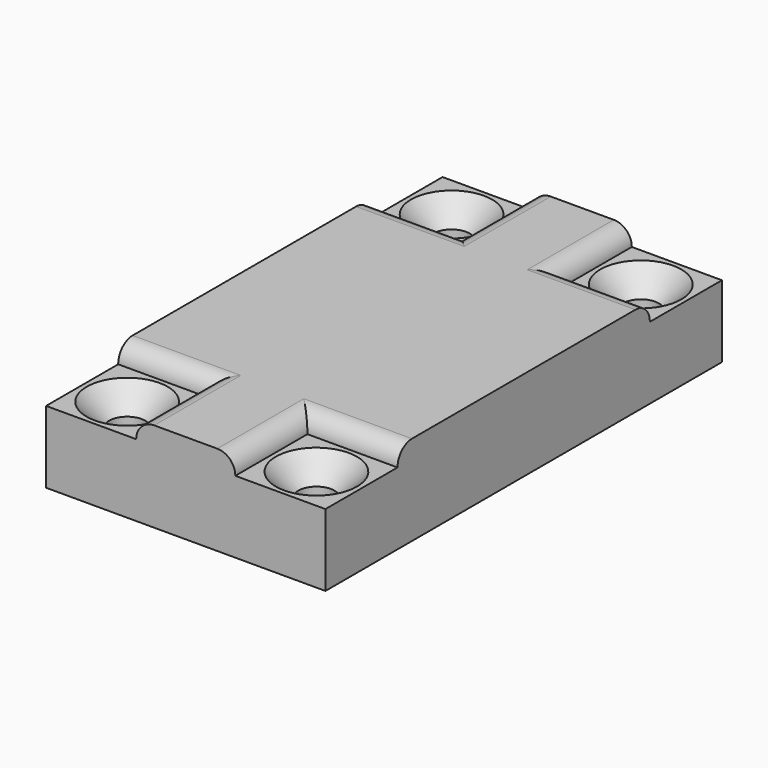
from build123d import *

# Parameters (mm, degrees)
F0_W     = 10
F0_H     = 18.5
F2_DEPTH = 10
F3_DEPTH = 3
F0_H_2   = 10
F4_DEPTH = 8
F1_R     = 2
F5_DEPTH = 25
F6_SIZE  = 2.5
F7_R     = 1.99999


# Not quite as in the source:
# - a fillet or chamfer is up to 0.001 mm smaller than in the source, because OpenCascade refuses the exact size


with BuildPart() as f2:
    # F0 (on Top) → F2 (new body)
    with BuildSketch(Plane.XY):
        with Locations((-10.5, 0.1457649022)):
            Rectangle(F0_W, F0_H)
        Polygon((5.5, 17.5), (5.5, 27.5), (-5.5, 27.5), (-5.5, 17.5), (-15.5, 17.5), (-15.5, 9.3957649022), (-5.5, 9.3957649022), (-5.5, -9.1042350978), (-15.5, -9.1042350978), (-15.5, -17.5), (-5.5, -17.5), (-5.5, -27.5), (5.5, -27.5), (5.5, -17.5), (15.5, -17.5), (15.5, 17.5), align=None)
    extrude(amount=F2_DEPTH)

    # F0 (on Top) → F3 (cut)
    with BuildSketch(Plane.XY):
        with Locations((-10.5, 0.1457649022)):
            Rectangle(F0_W, F0_H)
    extrude(amount=F3_DEPTH, mode=Mode.SUBTRACT)

    # F0 (on Top) → F4 (join)
    with BuildSketch(Plane.XY):
        with Locations((-10.5, 22.5)):
            Rectangle(F0_W, F0_H_2)
        with Locations((10.5, 22.5)):
            Rectangle(F0_W, F0_H_2)
        with Locations((-10.5, -22.5)):
            Rectangle(F0_W, F0_H_2)
        with Locations((10.5, -22.5)):
            Rectangle(F0_W, F0_H_2)
    extrude(amount=F4_DEPTH)

    # F1 (on Top) → F5 (cut)
    with BuildSketch(Plane.XY):
        with Locations((-10.4999503866, 22.4999412894)):
            Circle(F1_R)
        with Locations((10.4999503866, 22.4999412894)):
            Circle(F1_R)
        with Locations((-10.4999503866, -22.4999412894)):
            Circle(F1_R)
        with Locations((10.4999503866, -22.4999412894)):
            Circle(F1_R)
    extrude(amount=F5_DEPTH, mode=Mode.SUBTRACT)

    # F6
    f6_edges = [f2.edges().sort_by_distance(p)[0] for p in [
        (-12.49995, 22.499941, 8),
        (8.49995, 22.499941, 8),
        (8.49995, -22.499941, 8),
        (-12.49995, -22.499941, 8),
    ]]
    chamfer(f6_edges, length=F6_SIZE)

    # F7 (radius 2 in the source; OpenCascade refuses exactly that, so slightly less here)
    f7_edges = [f2.edges().sort_by_distance(p)[0] for p in [
        (-10.5, -17.5, 10),
        (-5.5, -22.5, 10),
        (-10.5, 17.5, 10),
        (-5.5, 22.5, 10),
        (5.5, 22.5, 10),
        (10.5, 17.5, 10),
        (10.5, -17.5, 10),
        (5.5, -22.5, 10),
    ]]
    fillet(f7_edges, radius=F7_R)


solid = f2.part
